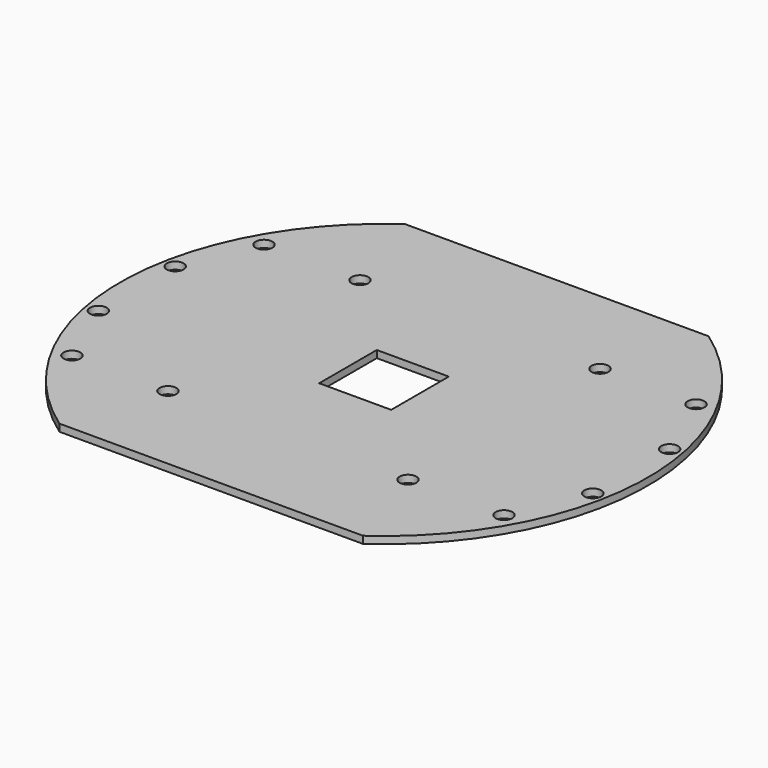
from build123d import *

# Parameters (mm, degrees)
F1_DEPTH = 3
F3_D     = 7
F5_D     = 7
F6_W     = 30
F6_H     = 30
F7_DEPTH = 3.001


# Not quite as in the source:
# - a feature names something its author has since deleted; it is built from what else it names


with BuildPart() as f1:
    # F0 (on Top) → F1 (new body)
    with BuildSketch(Plane.XY):
        with BuildLine():
            Line((63.2455532034, 90), (-63.2455532034, 90))
            ThreePointArc((-63.2455532034, 90), (-110, 0), (-63.2455532034, -90))
            Line((-63.2455532034, -90), (63.2455532034, -90))
            ThreePointArc((63.2455532034, -90), (110, 0), (63.2455532034, 90))
        make_face()
    extrude(amount=F1_DEPTH)

    # F3 (through all)
    with Locations(Plane.XY.offset(3)):
        with Locations((-103, 20), (-103, -20), (-90, 50), (-90, -50), (90, -50), (90, 50), (103, 20), (103, -20)):
            Hole(F3_D / 2)

    # F5 (through all)
    with Locations(Plane.XY.offset(3)):
        with Locations((-50, 50), (50, 50), (50, -50), (-50, -50)):
            Hole(F5_D / 2)

    # F6 (on face) → F7 (cut, through all)
    with BuildSketch(Plane.XY.offset(3)):
        Rectangle(F6_W, F6_H)
    extrude(amount=-F7_DEPTH, mode=Mode.SUBTRACT)


solid = f1.part
